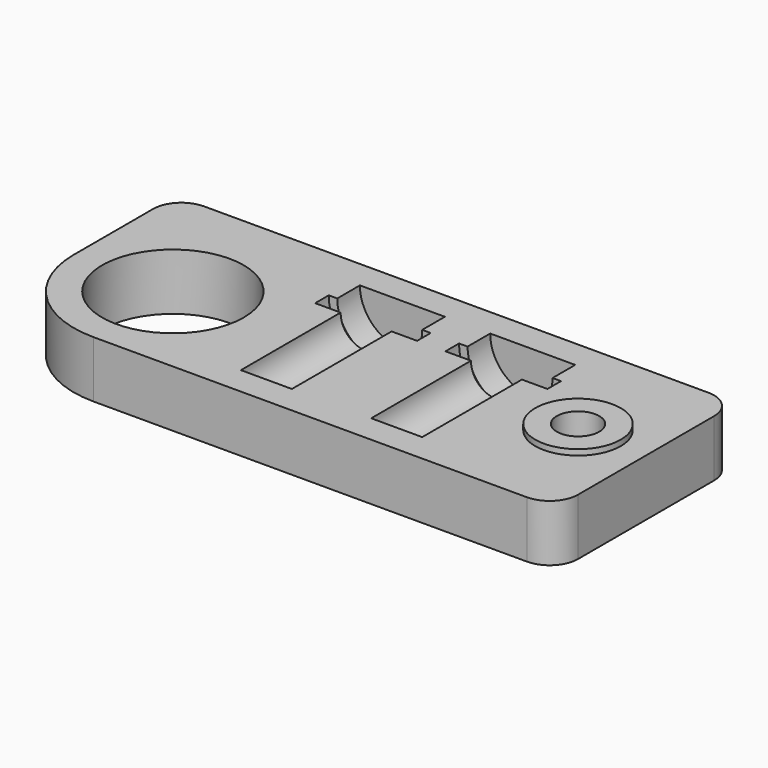
from build123d import *

# Parameters (mm, degrees)
F0_R         = 12.5
F1_DEPTH     = 10
F2_R         = 7.55
F2_R_2       = 3.75
F5_DEPTH     = 1
F6_DEPTH     = 9
F7_TEXT_SIZE = 5.5555555556
F8_DEPTH     = 1


# Not quite as in the source:
# - Text() gives the source's letters only with a copy of the font that has no kerning and outlines rounded to 1/6400 em; it was checked with that copy


with BuildPart() as f1:
    # F0 (on Top) → F1 (new body)
    with BuildSketch(Plane.XY):
        with BuildLine():
            ThreePointArc((0, 17.5), (5.1256313292, 5.1256313292), (17.5, 0))
            Line((17.5, 0), (94, 0))
            ThreePointArc((94, 0), (97.5355339059, 1.4644660941), (99, 5))
            Line((99, 5), (99, 35))
            ThreePointArc((99, 35), (97.5355339059, 38.5355339059), (94, 40))
            Line((94, 40), (5, 40))
            ThreePointArc((5, 40), (1.4644660941, 38.5355339059), (0, 35))
            Line((0, 35), (0, 17.5))
        make_face()
        with Locations((17.5, 17.5)):
            Circle(F0_R, mode=Mode.SUBTRACT)
    extrude(amount=F1_DEPTH)

    # F2 (on face) → F3 (revolve, cut)
    with BuildSketch(Plane.XY.offset(10)):
        Polygon((44, 27), (44, 5), (48.5, 5), (48.5, 27), (53, 27), (53, 30), (51.5, 30), (51.5, 35), (44, 35), (44, 30), align=None)
    revolve(axis=Axis((44, 16, 10), (0, 1, 0)), mode=Mode.SUBTRACT)

    # F2 (on face) → F4 (revolve, cut)
    with BuildSketch(Plane.XY.offset(10)):
        Polygon((67, 27), (67, 5), (71.5, 5), (71.5, 27), (76, 27), (76, 30), (74.5, 30), (74.5, 35), (67, 35), (67, 30), align=None)
    revolve(axis=Axis((67, 16, 10), (0, 1, 0)), mode=Mode.SUBTRACT)

    # F2 (on face) → F5 (join)
    with BuildSketch(Plane.XY.offset(10)):
        with Locations((87, 20)):
            Circle(F2_R)
        with Locations((87, 20)):
            Circle(F2_R_2, mode=Mode.SUBTRACT)
    extrude(amount=F5_DEPTH)

    # F2 (on face) → F6 (cut)
    with BuildSketch(Plane.XY.offset(10)):
        with Locations((87, 20)):
            Circle(F2_R_2)
    extrude(amount=-F6_DEPTH, mode=Mode.SUBTRACT)

    # F7 (on face) → F8 (cut)
    with BuildSketch(Plane(origin=(0, 0, 0), x_dir=(1, 0, 0), z_dir=(0, 0, -1))):
        with Locations((30, -9)):
            Text('813', F7_TEXT_SIZE, font='Open Sans', text_align=(TextAlign.LEFT, TextAlign.BOTTOM))
    extrude(amount=-F8_DEPTH, mode=Mode.SUBTRACT)


solid = f1.part
